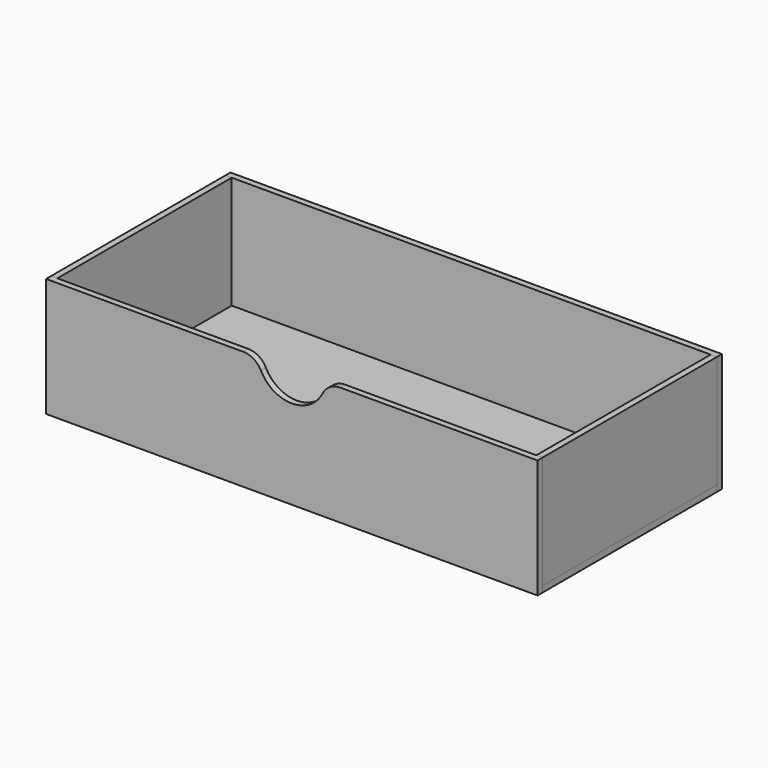
from build123d import *

# Parameters (mm, degrees)
F1_W      = 248
F1_H      = 60
F2_DEPTH  = 3.15
F3_R      = 17.5
F4_DEPTH  = 25
F5_R      = 10
F6_W      = 110
F6_H      = 56.85
F7_DEPTH  = 3.15
F9_W      = 248
F9_H      = 60
F10_DEPTH = 3.15
F11_W     = 248
F11_H     = 110
F12_DEPTH = 3.15


with BuildPart() as f2:
    # F1 (on Front) → F2 (new body)
    with BuildSketch(Plane.XZ):
        with Locations((124, 30)):
            Rectangle(F1_W, F1_H)
    extrude(amount=F2_DEPTH)

    # F3 (on face) → F4 (cut)
    with BuildSketch(Plane.XZ.offset(3.15)):
        with Locations((124, 62.5)):
            Circle(F3_R)
    extrude(amount=-F4_DEPTH, mode=Mode.SUBTRACT)

    # F5
    f5_edges = [f2.edges().sort_by_distance(p)[0] for p in [
        (106.679492, -1.575, 60),
        (141.320508, -1.575, 60),
    ]]
    fillet(f5_edges, radius=F5_R)


with BuildPart() as f7:
    # F6 (on face) → F7 (new body)
    with BuildSketch(Plane.YZ.offset(248)):
        with Locations((55, 31.575)):
            Rectangle(F6_W, F6_H)
    extrude(amount=-F7_DEPTH)


with BuildPart() as f8_1:
    # F8: copy of F7
    add(f7.part.moved(Location((-244.85, 0, 0))))


with BuildPart() as f10:
    # F9 (on face) → F10 (new body)
    with BuildSketch(Plane(origin=(0, 110, 0), x_dir=(-1, 0, 0), z_dir=(0, 1, 0))):
        with Locations((-124, 30)):
            Rectangle(F9_W, F9_H)
    extrude(amount=F10_DEPTH)


with BuildPart() as f12:
    # F11 (on face) → F12 (new body)
    with BuildSketch(Plane(origin=(0, 0, 3.15), x_dir=(1, 0, 0), z_dir=(0, 0, -1))):
        with Locations((124, -55)):
            Rectangle(F11_W, F11_H)
    extrude(amount=F12_DEPTH)


solid = Compound([f2.part, f7.part, f8_1.part, f10.part, f12.part])
